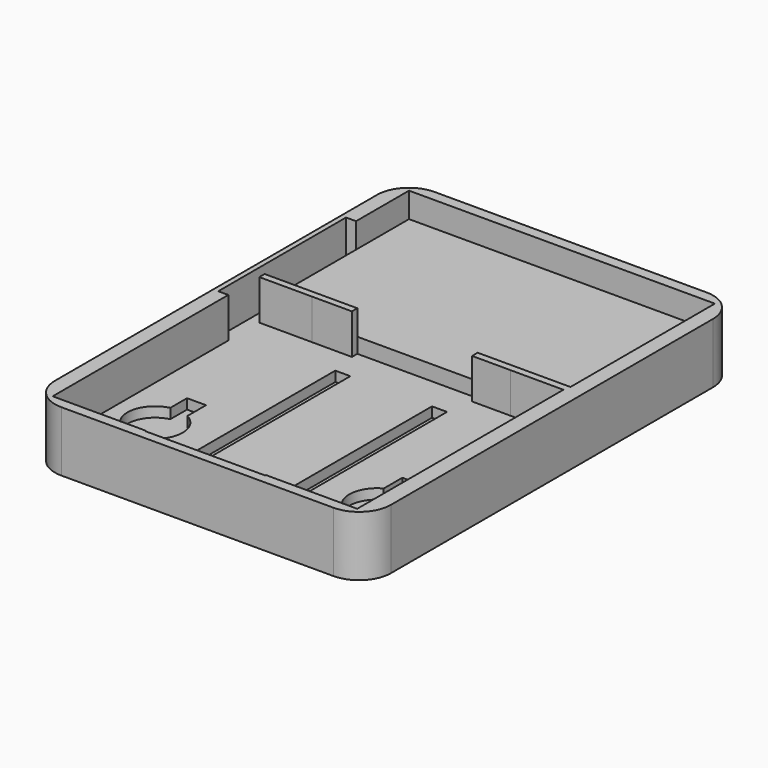
from build123d import *

# Parameters (mm, degrees)
F1_DEPTH = 12
F3_DEPTH = 5
F2_W     = 24
F2_H     = 53
F5_DEPTH = 8
F6_DEPTH = 10
F7_W     = 3
F7_H     = 40
F8_DEPTH = 10
F9_DEPTH = 10


with BuildPart() as f1:
    # F0 (on Top) → F1 (new body)
    with BuildSketch(Plane.XY):
        with BuildLine():
            Line((27.15, 46.5), (-27.15, 46.5))
            ThreePointArc((-27.15, 46.5), (-31.6401280605, 44.6401280605), (-33.5, 40.15))
            Line((-33.5, 40.15), (-33.5, -40.15))
            ThreePointArc((-33.5, -40.15), (-31.6401280605, -44.6401280605), (-27.15, -46.5))
            Line((-27.15, -46.5), (27.15, -46.5))
            ThreePointArc((27.15, -46.5), (31.6401280605, -44.6401280605), (33.5, -40.15))
            Line((33.5, -40.15), (33.5, 40.15))
            ThreePointArc((33.5, 40.15), (31.6401280605, 44.6401280605), (27.15, 46.5))
        make_face()
    extrude(amount=F1_DEPTH)

    # F2 (on face) → F3 (cut)
    with BuildSketch(Plane.XY.offset(12)):
        Polygon((-30.5, 31.1559867114), (-30.5, 8.3555228412), (-12, 8.3555228412), (12, 8.3555228412), (30.5, 8.3555228412), (30.5, 44.3555228412), (-30.5, 44.3555228412), align=None)
    extrude(amount=-F3_DEPTH, mode=Mode.SUBTRACT)

    # F4 (on face) + F2 (on face) → F5 (cut)
    with BuildSketch(Plane.XY.offset(12)):
        Polygon((-19.9947099381, 7.0137236979), (-30.5000375956, 7.0301252197), (-30.5000375956, -0.696099014), (-30.5000375956, -0.6988210371), (-30.5000375956, -44.4698496722), (-12, -44.4698496722), (-12, 7.0012418968), align=None)
        with BuildLine():
            Line((-19.57828179, -19.8942141583), (-19.57828179, -24.546026914))
            ThreePointArc((-19.57828179, -24.546026914), (-17.4189463665, -26.5711645765), (-16.6222270916, -29.4223310783))
            ThreePointArc((-16.6222270916, -29.4223310783), (-25.5439247807, -33.7283715941), (-23.364767064, -24.064524212))
            Line((-23.364767064, -24.064524212), (-23.364767064, -19.8942141583))
            Line((-23.364767064, -19.8942141583), (-19.57828179, -19.8942141583))
        make_face(mode=Mode.SUBTRACT)
        Polygon((19.6427109083, 6.9518394763), (12, 6.9637717162), (12, -44.4698496722), (30.2305370569, -44.4698496722), (30.2305370569, 6.9353091531), align=None)
        with BuildLine():
            Line((23.364767064, -19.8942141583), (23.364767064, -24.064524212))
            ThreePointArc((23.364767064, -24.064524212), (26.4282676075, -26.0006333892), (27.6222270916, -29.4223310783))
            ThreePointArc((27.6222270916, -29.4223310783), (19.2710605898, -34.1256118034), (19.57828179, -24.546026914))
            Line((19.57828179, -24.546026914), (19.57828179, -19.8942141583))
            Line((19.57828179, -19.8942141583), (23.364767064, -19.8942141583))
        make_face(mode=Mode.SUBTRACT)
    with BuildSketch(Plane.XY.offset(12)):
        Polygon((-30.5, -0.696099014), (-30.5, 8.3555228412), (-30.5, 31.1559867114), (-32.5, 31.1559867114), (-32.5, -0.696099014), align=None)
        with Locations((0, -18.1444771588)):
            Rectangle(F2_W, F2_H)
        with BuildLine():
            ThreePointArc((-23.364767064, -24.064524212), (-21.4284150344, -23.9662679528), (-19.57828179, -24.546026914))
            Line((-19.57828179, -24.546026914), (-19.57828179, -19.8942141583))
            Line((-19.57828179, -19.8942141583), (-23.364767064, -19.8942141583))
            Line((-23.364767064, -19.8942141583), (-23.364767064, -24.064524212))
        make_face()
        with BuildLine():
            ThreePointArc((19.57828179, -24.546026914), (21.4284150344, -23.9662679528), (23.364767064, -24.064524212))
            Line((23.364767064, -24.064524212), (23.364767064, -19.8942141583))
            Line((23.364767064, -19.8942141583), (19.57828179, -19.8942141583))
            Line((19.57828179, -19.8942141583), (19.57828179, -24.546026914))
        make_face()
    extrude(amount=-F5_DEPTH, mode=Mode.SUBTRACT)

    # F2 (on face) → F6 (cut)
    with BuildSketch(Plane.XY.offset(12)):
        with BuildLine():
            ThreePointArc((-23.364767064, -24.064524212), (-25.5439247807, -33.7283715941), (-16.6222270916, -29.4223310783))
            ThreePointArc((-16.6222270916, -29.4223310783), (-17.4189463665, -26.5711645765), (-19.57828179, -24.546026914))
            ThreePointArc((-19.57828179, -24.546026914), (-21.4284150344, -23.9662679528), (-23.364767064, -24.064524212))
        make_face()
        with BuildLine():
            ThreePointArc((19.57828179, -24.546026914), (19.2710605898, -34.1256118034), (27.6222270916, -29.4223310783))
            ThreePointArc((27.6222270916, -29.4223310783), (26.4282676075, -26.0006333892), (23.364767064, -24.064524212))
            ThreePointArc((23.364767064, -24.064524212), (21.4284150344, -23.9662679528), (19.57828179, -24.546026914))
        make_face()
    extrude(amount=-F6_DEPTH, mode=Mode.SUBTRACT)

    # F7 (on face) → F8 (cut)
    with BuildSketch(Plane.XY.offset(12)):
        with Locations((-9.6433593556, -18.214944303)):
            Rectangle(F7_W, F7_H)
        Polygon((8.1433593556, 1.785055697), (8.1433593556, -38.214944303), (9.8566406444, -38.214944303), (11.1433593556, -38.214944303), (11.1433593556, 1.785055697), align=None)
    extrude(amount=-F8_DEPTH, mode=Mode.SUBTRACT)

    # F4 (on face) + F2 (on face) → F9 (cut)
    with BuildSketch(Plane.XY.offset(12)):
        with BuildLine():
            ThreePointArc((-16.6222270916, -29.4223310783), (-17.4189463665, -26.5711645765), (-19.57828179, -24.546026914))
            Line((-19.57828179, -24.546026914), (-19.57828179, -19.8942141583))
            Line((-19.57828179, -19.8942141583), (-23.364767064, -19.8942141583))
            Line((-23.364767064, -19.8942141583), (-23.364767064, -24.064524212))
            ThreePointArc((-23.364767064, -24.064524212), (-25.5439247807, -33.7283715941), (-16.6222270916, -29.4223310783))
        make_face()
    with BuildSketch(Plane.XY.offset(12)):
        with BuildLine():
            ThreePointArc((19.57828179, -24.546026914), (19.2710605898, -34.1256118034), (27.6222270916, -29.4223310783))
            ThreePointArc((27.6222270916, -29.4223310783), (26.4282676075, -26.0006333892), (23.364767064, -24.064524212))
            ThreePointArc((23.364767064, -24.064524212), (21.4284150344, -23.9662679528), (19.57828179, -24.546026914))
        make_face()
        with BuildLine():
            ThreePointArc((19.57828179, -24.546026914), (21.4284150344, -23.9662679528), (23.364767064, -24.064524212))
            Line((23.364767064, -24.064524212), (23.364767064, -19.8942141583))
            Line((23.364767064, -19.8942141583), (19.57828179, -19.8942141583))
            Line((19.57828179, -19.8942141583), (19.57828179, -24.546026914))
        make_face()
    extrude(amount=-F9_DEPTH, mode=Mode.SUBTRACT)


solid = f1.part
